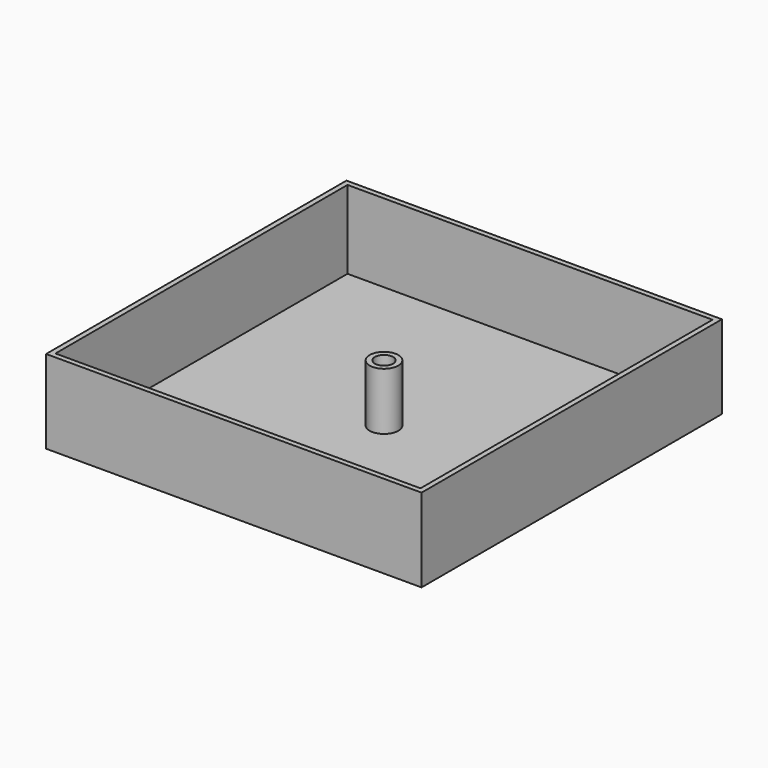
from build123d import *

# Parameters (mm, degrees)
F0_W         = 72
F0_H         = 72
F1_DEPTH     = 1
F2_R         = 2.75
F2_R_2       = 1.75
F3_DEPTH     = 11
F4_W         = 70
F4_H         = 1
F5_DEPTH     = 15
F6_R         = 1.75
F7_DEPTH     = 6
F8_TEXT_SIZE = 13.8888888889
F9_DEPTH     = 0.4


# Not quite as in the source:
# - Text() gives the source's letters only with a copy of the font that has no kerning and outlines rounded to 1/6400 em; it was checked with that copy


with BuildPart() as f1:
    # F0 (on Top) → F1 (new body)
    with BuildSketch(Plane.XY):
        Rectangle(F0_W, F0_H)
    extrude(amount=F1_DEPTH)

    # F2 (on face) → F3 (join)
    with BuildSketch(Plane.XY.offset(1)):
        Circle(F2_R)
        Circle(F2_R_2, mode=Mode.SUBTRACT)
    extrude(amount=F3_DEPTH)

    # F4 (on face) → F5 (join)
    with BuildSketch(Plane.XY.offset(1)):
        Polygon((-35, 36), (-36, 36), (-36, -36), (-35, -36), (-35, -35), (-35, 35), align=None)
        with Locations((0, 35.5)):
            Rectangle(F4_W, F4_H)
        Polygon((36, 36), (35, 36), (35, 35), (35, -35), (35, -36), (36, -36), align=None)
        with Locations((0, -35.5)):
            Rectangle(F4_W, F4_H)
    extrude(amount=F5_DEPTH)

    # F6 (on face) → F7 (join)
    with BuildSketch(Plane.XY.offset(1)):
        Circle(F6_R)
    extrude(amount=F7_DEPTH)

    # F8 (on face) → F9 (cut)
    with BuildSketch(Plane(origin=(0, 0, 0), x_dir=(1, 0, 0), z_dir=(0, 0, -1))):
        with Locations((-24.0505642361, -31)):
            Text('Button', F8_TEXT_SIZE, font='Open Sans', font_style=FontStyle.BOLD, text_align=(TextAlign.LEFT, TextAlign.BOTTOM))
    extrude(amount=-F9_DEPTH, mode=Mode.SUBTRACT)


solid = f1.part
